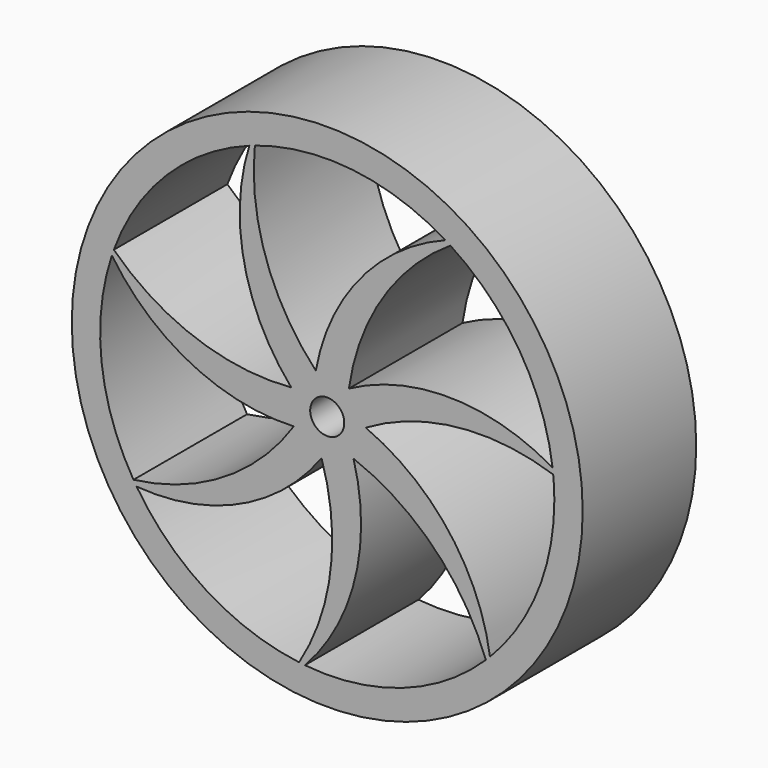
from build123d import *

# Parameters (mm, degrees)
F0_R     = 45
F0_R_2   = 3
F1_DEPTH = 25
F2_COUNT = 7


# Not quite as in the source:
# - a feature names something its author has since deleted; it is built from what else it names


with BuildPart() as f1:
    # F0 (on Front) → F1 (new body)
    with BuildSketch(Plane.XZ):
        Circle(F0_R)
        with BuildLine():
            ThreePointArc((40, 0), (-34.8753984239, -19.58842987), (20.8146707615, 34.1577148107))
            ThreePointArc((20.8146707615, 34.1577148107), (21.2557560399, 33.8849942478), (21.693268588, 33.6065781949))
            ThreePointArc((21.693268588, 33.6065781949), (35.126419854, 19.1346447116), (40, 0))
        make_face(mode=Mode.SUBTRACT)
        with BuildLine():
            ThreePointArc((20.8146707615, 34.1577148107), (4.7404997755, 21.9880977011), (-2.457993575, 3.1556722874))
            ThreePointArc((-2.457993575, 3.1556722874), (-0.7771850997, -3.9237715684), (3.4753115022, 1.9804570085))
            ThreePointArc((3.4753115022, 1.9804570085), (8.7719800119, 19.9895662469), (21.693268588, 33.6065781949))
            ThreePointArc((21.693268588, 33.6065781949), (21.2557560399, 33.8849942478), (20.8146707615, 34.1577148107))
        make_face()
        Circle(F0_R_2, mode=Mode.SUBTRACT)
    extrude(amount=F1_DEPTH)

    # F2: F1 ×7 about axis
    f2_axis = Axis((0, -25, 0), (0, -1, 0))


with BuildPart() as f1_1:
    add(f1.part)
    for i in range(1, F2_COUNT):
        add(f1.part.rotate(f2_axis, i * 360 / F2_COUNT))


solid = f1_1.part
